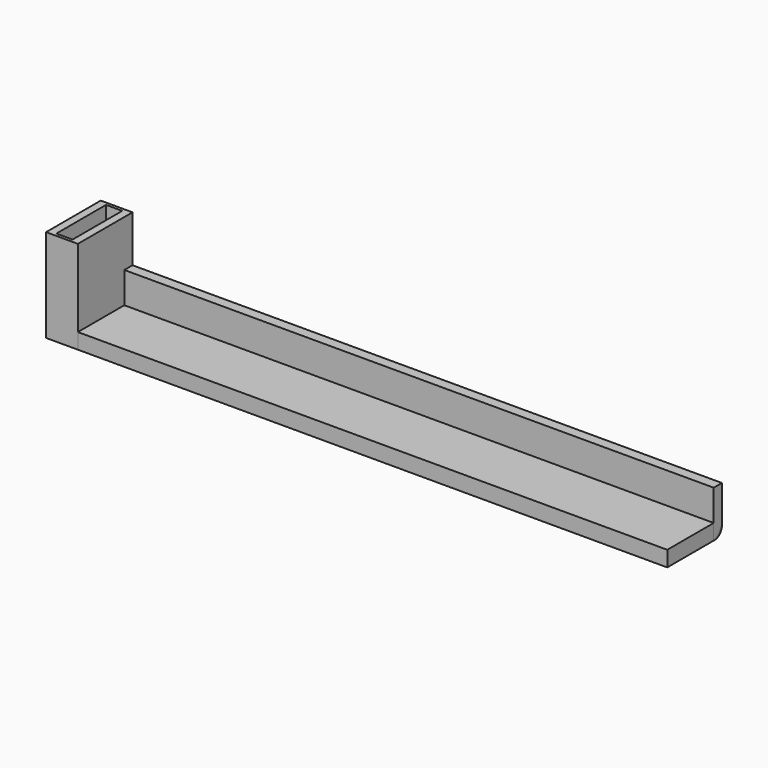
from build123d import *

# Parameters (mm, degrees)
F0_W          = 5.2268145978
F0_H          = 17.7
F0_H_2        = 2.3
F0_W_2        = 2.5
F1_DEPTH      = 5
F2_DEPTH      = 30
F3_DEPTH      = 15
F4_T1_DEPTH   = 35.2268145978
F4_2_T1_DEPTH = 213.2838212932
F5_R          = 3


# Not quite as in the source:
# - a fillet or chamfer that OpenCascade refuses, or shapes differently, is made with other operations: its cross-section is extruded or revolved along the edge and cut away or added


with BuildPart() as f1:
    # F0 (on Top) → F1 (new body)
    with BuildSketch(Plane.XY):
        with Locations((-37.1891043335, 19.0716543853)):
            Rectangle(F0_W, F0_H)
        Polygon((157.6974883676, 9.2216543853), (157.6974883676, 27.9216543853), (-32.0756970346, 27.9216543853), (-32.0756970346, 10.2216543853), (-32.0756970346, 9.2216543853), align=None)
        with Locations((-37.1891043335, 29.0716543853)):
            Rectangle(F0_W, F0_H_2)
        Polygon((-39.8025116324, 10.2216543853), (-42.3025116324, 10.2216543853), (-42.3025116324, 9.2216543853), (-32.0756970346, 9.2216543853), (-32.0756970346, 10.2216543853), (-34.5756970346, 10.2216543853), align=None)
        with Locations((-33.3256970346, 19.0716543853)):
            Rectangle(F0_W_2, F0_H)
        with Locations((-41.0525116324, 19.0716543853)):
            Rectangle(F0_W_2, F0_H)
        with Locations((-41.0525116324, 29.0716543853)):
            Rectangle(F0_W_2, F0_H_2)
        Polygon((-32.0756970346, 31.2216543853), (-42.3025116324, 31.2216543853), (-42.3025116324, 30.2216543853), (-39.8025116324, 30.2216543853), (-34.5756970346, 30.2216543853), (-32.0756970346, 30.2216543853), align=None)
        with Locations((-33.3256970346, 29.0716543853)):
            Rectangle(F0_W_2, F0_H_2)
        Polygon((157.6974883676, 31.2216543853), (-32.0756970346, 31.2216543853), (-32.0756970346, 30.2216543853), (-32.0756970346, 27.9216543853), (157.6974883676, 27.9216543853), align=None)
    extrude(amount=F1_DEPTH)

    # F5
    f5_edges = [f1.edges().sort_by_distance(p)[0] for p in [
        (57.697488, 31.221654, 0),
    ]]
    fillet(f5_edges, radius=F5_R)


with BuildPart() as f2:
    # F0 (on Top) → F2 (new body)
    with BuildSketch(Plane.XY):
        Polygon((-32.0756970346, 31.2216543853), (-42.3025116324, 31.2216543853), (-42.3025116324, 30.2216543853), (-39.8025116324, 30.2216543853), (-34.5756970346, 30.2216543853), (-32.0756970346, 30.2216543853), align=None)
        with Locations((-33.3256970346, 29.0716543853)):
            Rectangle(F0_W_2, F0_H_2)
        with Locations((-33.3256970346, 19.0716543853)):
            Rectangle(F0_W_2, F0_H)
        with Locations((-41.0525116324, 29.0716543853)):
            Rectangle(F0_W_2, F0_H_2)
        with Locations((-41.0525116324, 19.0716543853)):
            Rectangle(F0_W_2, F0_H)
        Polygon((-39.8025116324, 10.2216543853), (-42.3025116324, 10.2216543853), (-42.3025116324, 9.2216543853), (-32.0756970346, 9.2216543853), (-32.0756970346, 10.2216543853), (-34.5756970346, 10.2216543853), align=None)
    extrude(amount=F2_DEPTH)

    # F4: fillet of radius 5 on 1 edges, made by hand

    # F4_s2 → F4_t1 (cut)
    with BuildSketch(Plane.YZ.offset(-54.8025116324)):
        with BuildLine():
            ThreePointArc((31.2216543853, 5), (29.7571882913, 1.4644660941), (26.2216543853, 0))
            Line((26.2216543853, 0), (31.2216543853, 0))
            Line((31.2216543853, 0), (31.2216543853, 5))
        make_face()
    extrude(amount=F4_T1_DEPTH, mode=Mode.SUBTRACT)


with BuildPart() as f3:
    # F0 (on Top) → F3 (new body)
    with BuildSketch(Plane.XY):
        Polygon((157.6974883676, 31.2216543853), (-32.0756970346, 31.2216543853), (-32.0756970346, 30.2216543853), (-32.0756970346, 27.9216543853), (157.6974883676, 27.9216543853), align=None)
    extrude(amount=F3_DEPTH)

    # F4#2: fillet of radius 5 on 1 edges, made by hand

    # F4_2_s2 → F4_2_t1 (cut)
    with BuildSketch(Plane.YZ.offset(-43.8310149801)):
        with BuildLine():
            ThreePointArc((31.2216543853, 4.7021271782), (30.3143307713, 1.8298458549), (27.9216543853, 0))
            Line((27.9216543853, 0), (31.2216543853, 0))
            Line((31.2216543853, 0), (31.2216543853, 4.7021271782))
        make_face()
    extrude(amount=F4_2_T1_DEPTH, mode=Mode.SUBTRACT)


solid = Compound([f1.part, f2.part, f3.part])
